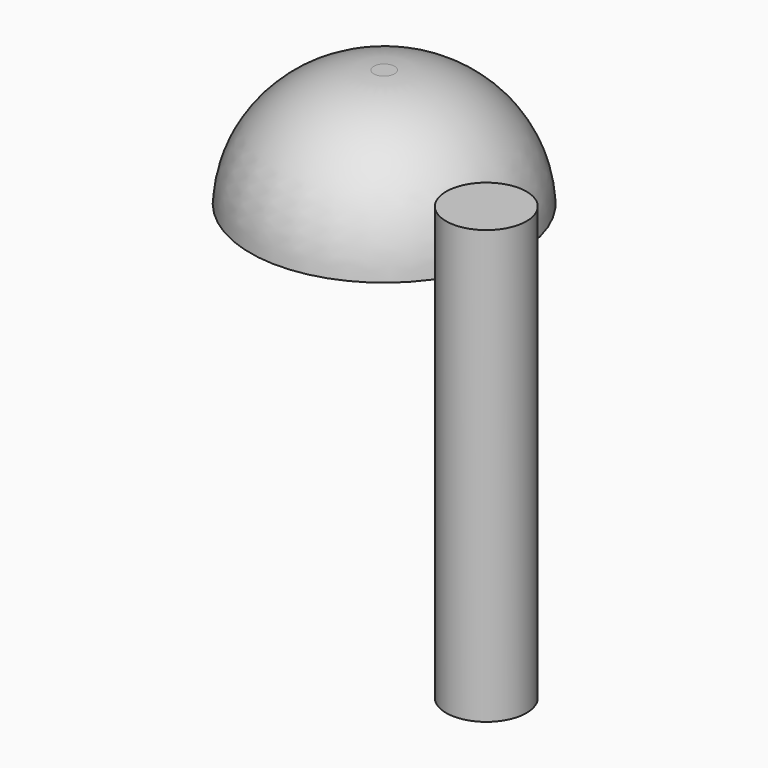
from build123d import *

# Parameters (mm, degrees)
F0_R     = 1.651
F1_DEPTH = 17.78
F2_R     = 5.4991
F3_DEPTH = 4.826
F4_R     = 5.4087768166
F5_DEPTH = 2.54
F6_R     = 2.53999


# Not quite as in the source:
# - a fillet or chamfer that OpenCascade refuses, or shapes differently, is made with other operations: its cross-section is extruded or revolved along the edge and cut away or added
# - a fillet or chamfer is up to 0.001 mm smaller than in the source, because OpenCascade refuses the exact size


with BuildPart() as f1:
    # F0 (on Top) → F1 (new body)
    with BuildSketch(Plane.XY):
        with Locations((-38.9938168228, 23.95244129)):
            Circle(F0_R)
    extrude(amount=F1_DEPTH)


with BuildPart() as f3:
    # F2 (on Top) → F3 (new body)
    with BuildSketch(Plane.XY):
        with Locations((-63.0094558001, 48.7264692783)):
            Circle(F2_R)
    extrude(amount=F3_DEPTH)

    # F4 (on face) → F5 (cut)
    with BuildSketch(Plane(origin=(0, 0, 0), x_dir=(1, 0, 0), z_dir=(0, 0, -1))):
        with Locations((-63.0094558001, -48.7264692783)):
            Circle(F4_R)
    extrude(amount=-F5_DEPTH, mode=Mode.SUBTRACT)

    # F6 (radius 2.54 in the source; OpenCascade refuses exactly that, so slightly less here)
    f6_edges = [f3.edges().sort_by_distance(p)[0] for p in [
        (-68.418233, 48.726469, 2.54),
    ]]
    fillet(f6_edges, radius=F6_R)

    # F7: fillet of radius 5.08 on 1 edges, made by hand

    # F7_s1 → F7_t2 (revolve, cut)
    with BuildSketch(Plane.XZ.offset(-48.7264692783)):
        with BuildLine():
            ThreePointArc((-57.5103558001, 0), (-59.0828534433, 3.4268096935), (-62.5840018263, 4.826))
            Line((-62.5840018263, 4.826), (-57.5103558001, 4.826))
            Line((-57.5103558001, 4.826), (-57.5103558001, 0))
        make_face()
    revolve(axis=Axis((-63.0094558001, 48.7264692783, 4.826), (0, 0, 1)), mode=Mode.SUBTRACT)


solid = Compound([f1.part, f3.part])
